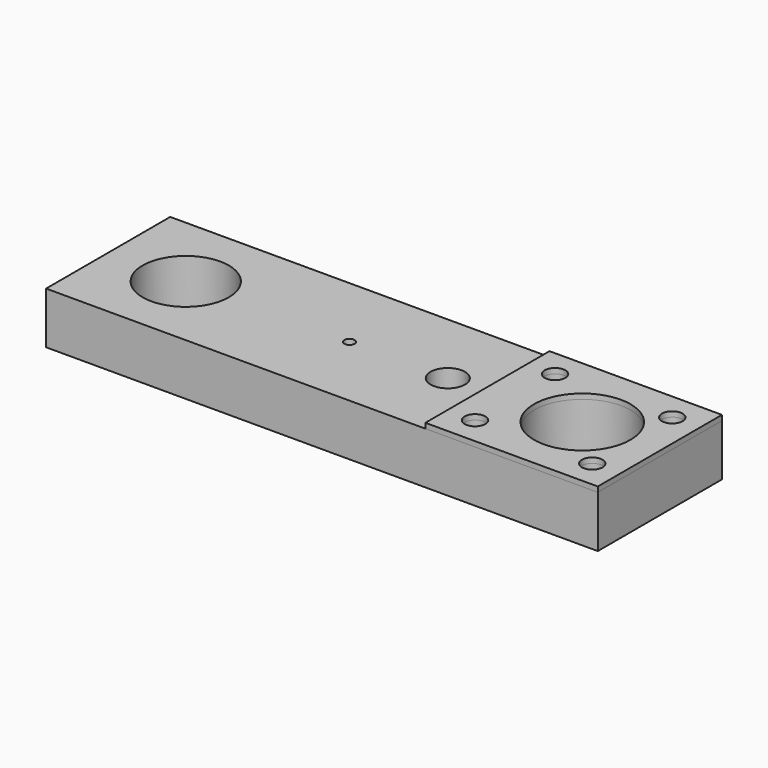
from build123d import *

# Parameters (mm, degrees)
F0_W     = 160
F0_H     = 45
F0_R     = 6
F0_R_2   = 12.5
F0_R_3   = 10
F0_R_4   = 14
F0_R_5   = 5
F0_R_6   = 3
F1_DEPTH = 15
F2_DEPTH = 5
F3_DEPTH = 9
F4_R     = 1.5
F5_DEPTH = 10
F6_W     = 50
F6_H     = 45
F6_R     = 3
F6_R_2   = 14
F7_DEPTH = 1.5


# Not quite as in the source:
# - a feature names something its author has since deleted; it is built from what else it names


with BuildPart() as f1:
    # F0 (on Top) → F1 (new body)
    with BuildSketch(Plane.XY):
        Rectangle(F0_W, F0_H)
        with Locations((38, -14.5)):
            Circle(F0_R, mode=Mode.SUBTRACT)
        with Locations((72, -14.5)):
            Circle(F0_R, mode=Mode.SUBTRACT)
        with Locations((-57.5, 0)):
            Circle(F0_R_2, mode=Mode.SUBTRACT)
        with Locations((18.5, 0)):
            Circle(F0_R_3, mode=Mode.SUBTRACT)
        with Locations((57.5, 0)):
            Circle(F0_R_4, mode=Mode.SUBTRACT)
        with Locations((38, 14.5)):
            Circle(F0_R, mode=Mode.SUBTRACT)
        with Locations((72, 14.5)):
            Circle(F0_R, mode=Mode.SUBTRACT)
        with Locations((18.5, 0)):
            Circle(F0_R_3)
        with Locations((18.5, 0)):
            Circle(F0_R_5, mode=Mode.SUBTRACT)
        with Locations((38, -14.5)):
            Circle(F0_R)
        with Locations((38, -14.5)):
            Circle(F0_R_6, mode=Mode.SUBTRACT)
        with Locations((72, -14.5)):
            Circle(F0_R)
        with Locations((72, -14.5)):
            Circle(F0_R_6, mode=Mode.SUBTRACT)
        with Locations((72, 14.5)):
            Circle(F0_R)
        with Locations((72, 14.5)):
            Circle(F0_R_6, mode=Mode.SUBTRACT)
        with Locations((38, 14.5)):
            Circle(F0_R)
        with Locations((38, 14.5)):
            Circle(F0_R_6, mode=Mode.SUBTRACT)
    extrude(amount=F1_DEPTH)

    # F0 (on Top) → F2 (cut)
    with BuildSketch(Plane.XY):
        with Locations((18.5, 0)):
            Circle(F0_R_3)
        with Locations((18.5, 0)):
            Circle(F0_R_5, mode=Mode.SUBTRACT)
    extrude(amount=F2_DEPTH, mode=Mode.SUBTRACT)

    # F0 (on Top) → F3 (cut)
    with BuildSketch(Plane.XY):
        with Locations((38, -14.5)):
            Circle(F0_R)
        with Locations((38, -14.5)):
            Circle(F0_R_6, mode=Mode.SUBTRACT)
        with Locations((72, -14.5)):
            Circle(F0_R)
        with Locations((72, -14.5)):
            Circle(F0_R_6, mode=Mode.SUBTRACT)
        with Locations((72, 14.5)):
            Circle(F0_R)
        with Locations((72, 14.5)):
            Circle(F0_R_6, mode=Mode.SUBTRACT)
        with Locations((38, 14.5)):
            Circle(F0_R)
        with Locations((38, 14.5)):
            Circle(F0_R_6, mode=Mode.SUBTRACT)
    extrude(amount=F3_DEPTH, mode=Mode.SUBTRACT)

    # F4 (on face) → F5 (cut)
    with BuildSketch(Plane.XY.offset(15)):
        with Locations((-10, 0)):
            Circle(F4_R)
    extrude(amount=-F5_DEPTH, mode=Mode.SUBTRACT)


with BuildPart() as f7:
    # F6 (on face) → F7 (new body)
    with BuildSketch(Plane.XY.offset(15)):
        with Locations((55, 0)):
            Rectangle(F6_W, F6_H)
        with Locations((38, -14.5)):
            Circle(F6_R, mode=Mode.SUBTRACT)
        with Locations((72, -14.5)):
            Circle(F6_R, mode=Mode.SUBTRACT)
        with Locations((57.5, 0)):
            Circle(F6_R_2, mode=Mode.SUBTRACT)
        with Locations((38, 14.5)):
            Circle(F6_R, mode=Mode.SUBTRACT)
        with Locations((72, 14.5)):
            Circle(F6_R, mode=Mode.SUBTRACT)
    extrude(amount=F7_DEPTH)


solid = Compound([f1.part, f7.part])
